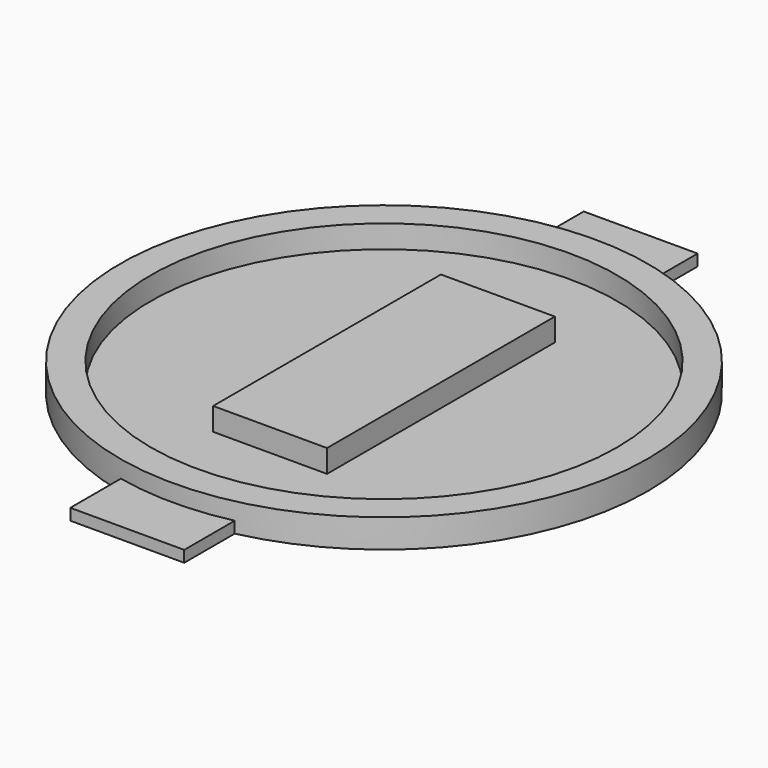
from build123d import *

# Parameters (mm, degrees)
F0_R     = 46.35
F1_DEPTH = 5
F2_R     = 40.9537225283
F2_W     = 20
F2_H     = 50
F3_DEPTH = 4
F5_DEPTH = 2
F6_DEPTH = 2


# Not quite as in the source:
# - a feature names something its author has since deleted; it is built from what else it names


with BuildPart() as f1:
    # F0 (on Top) → F1 (new body)
    with BuildSketch(Plane.XY):
        Circle(F0_R)
    extrude(amount=F1_DEPTH)

    # F2 (on face) → F3 (cut)
    with BuildSketch(Plane.XY.offset(5)):
        Circle(F2_R)
        Rectangle(F2_W, F2_H, mode=Mode.SUBTRACT)
    extrude(amount=-F3_DEPTH, mode=Mode.SUBTRACT)

    # F4 (on face) → F5 (join)
    with BuildSketch(Plane.XY):
        with BuildLine():
            Line((10, 45.2583970109), (10, 56.35))
            Line((10, 56.35), (0, 56.35))
            Line((0, 56.35), (-10, 56.35))
            Line((-10, 56.35), (-10, 45.2583970109))
            ThreePointArc((-10, 45.2583970109), (0, 46.35), (10, 45.2583970109))
        make_face()
    extrude(amount=F5_DEPTH)

    # F4 (on face) → F6 (join)
    with BuildSketch(Plane.XY):
        with BuildLine():
            Line((10, -56.35), (10, -45.2583970109))
            ThreePointArc((10, -45.2583970109), (0, -46.35), (-10, -45.2583970109))
            Line((-10, -45.2583970109), (-10, -56.35))
            Line((-10, -56.35), (10, -56.35))
        make_face()
    extrude(amount=F6_DEPTH)


solid = f1.part
